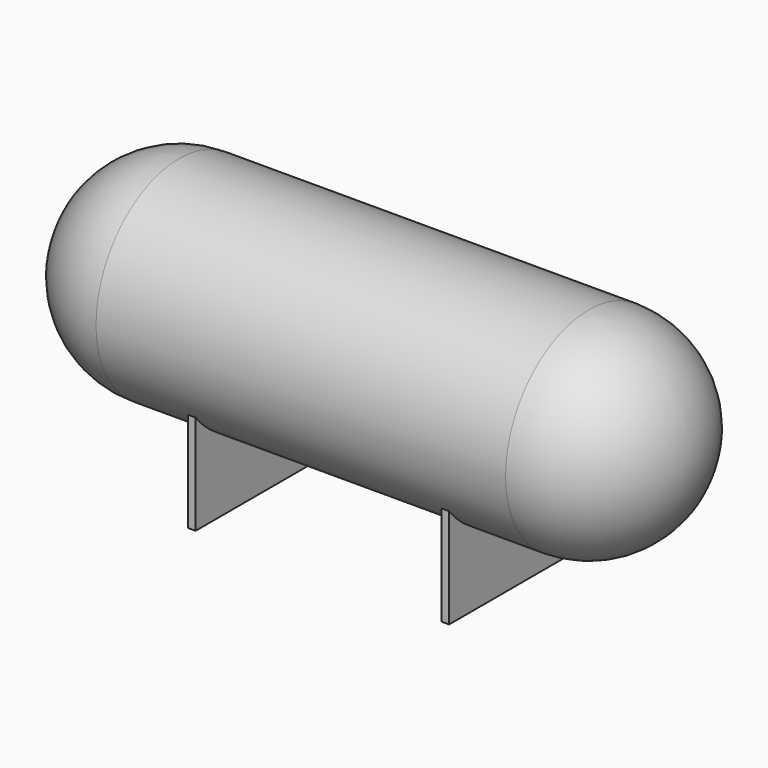
from build123d import *

# Parameters (mm, degrees)
F4_DEPTH = 19.05


# Not quite as in the source:
# - a length typed as a fraction of an inch, garbled in the dataset ("3 / 203.2 mm" for 3/8 in), is restored


with BuildPart() as f1:
    # F0 (on Front) → F1 (revolve)
    with BuildSketch(Plane.XZ):
        with BuildLine():
            Line((-754, 0), (-750, 0))
            ThreePointArc((-750, 0), (-676.7766952966, 176.7766952966), (-500, 250))
            Line((-500, 250), (0, 250))
            Line((0, 250), (500, 250))
            ThreePointArc((500, 250), (676.7766952966, 176.7766952966), (750, 0))
            Line((750, 0), (754, 0))
            ThreePointArc((754, 0), (679.6051224214, 179.6051224214), (500, 254))
            Line((500, 254), (0, 254))
            Line((0, 254), (-500, 254))
            ThreePointArc((-500, 254), (-679.6051224214, 179.6051224214), (-754, 0))
        make_face()
    revolve(axis=Axis((-250, 0, 0), (-1, 0, 0)))

    # F3 (on offset) → F4 (join)
    with BuildSketch(Plane.YZ.offset(300)):
        with BuildLine():
            ThreePointArc((200, -156.5758602084), (0, -254), (-200, -156.5758602084))
            Line((-200, -156.5758602084), (-200, -400))
            Line((-200, -400), (200, -400))
            Line((200, -400), (200, -156.5758602084))
        make_face()
    extrude(amount=F4_DEPTH)

    # F5: F1 across plane


with BuildPart() as f1_1:
    add(f1.part)
    add(f1.part.mirror(Plane.YZ))


solid = f1_1.part
